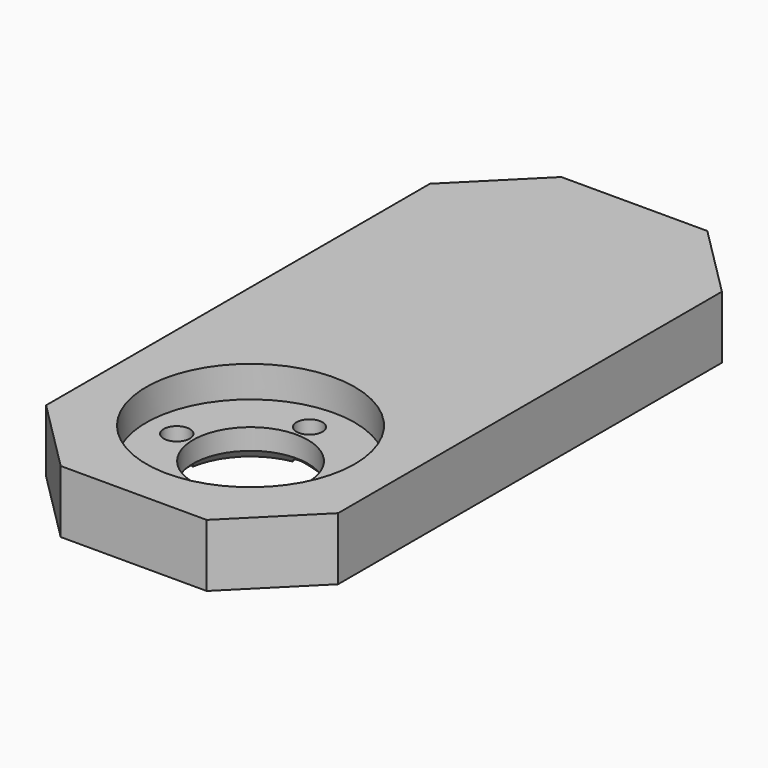
from build123d import *

# Parameters (mm, degrees)
F0_W     = 28
F0_H     = 60
F1_DEPTH = 6
F2_R     = 10
F3_DEPTH = 3
F4_R     = 5.5
F4_R_2   = 1.25
F5_DEPTH = 3.001
F7_SIZE  = 7


# Not quite as in the source:
# - a fillet or chamfer that OpenCascade refuses, or shapes differently, is made with other operations: its cross-section is extruded or revolved along the edge and cut away or added


with BuildPart() as f1:
    # F0 (on Top) → F1 (new body)
    with BuildSketch(Plane.XY):
        with Locations((0, 16)):
            Rectangle(F0_W, F0_H)
    extrude(amount=F1_DEPTH)

    # F2 (on face) → F3 (cut)
    with BuildSketch(Plane.XY.offset(6)):
        Circle(F2_R)
    extrude(amount=-F3_DEPTH, mode=Mode.SUBTRACT)

    # F4 (on face) → F5 (cut, through all)
    with BuildSketch(Plane.XY.offset(3)):
        Circle(F4_R)
        with Locations((0, 7.0710678119)):
            Circle(F4_R_2)
        with Locations((7.0710678119, 0)):
            Circle(F4_R_2)
        with Locations((0, -7.0710678119)):
            Circle(F4_R_2)
        with Locations((-7.0710678119, 0)):
            Circle(F4_R_2)
    extrude(amount=-F5_DEPTH, mode=Mode.SUBTRACT)

    # F6: chamfer of 1 on 1 edges, made by hand

    # F6_s1 → F6_t2 (revolve, cut)
    with BuildSketch(Plane.XZ):
        Polygon((6.5, 0), (5.5, 1), (5.5, 0), align=None)
    revolve(axis=Axis((0, 0, 0), (0, 0, 1)), mode=Mode.SUBTRACT)

    # F7
    f7_edges = [f1.edges().sort_by_distance(p)[0] for p in [
        (14, -14, 3),
        (-14, -14, 3),
        (14, 46, 3),
        (-14, 46, 3),
    ]]
    chamfer(f7_edges, length=F7_SIZE)


solid = f1.part
